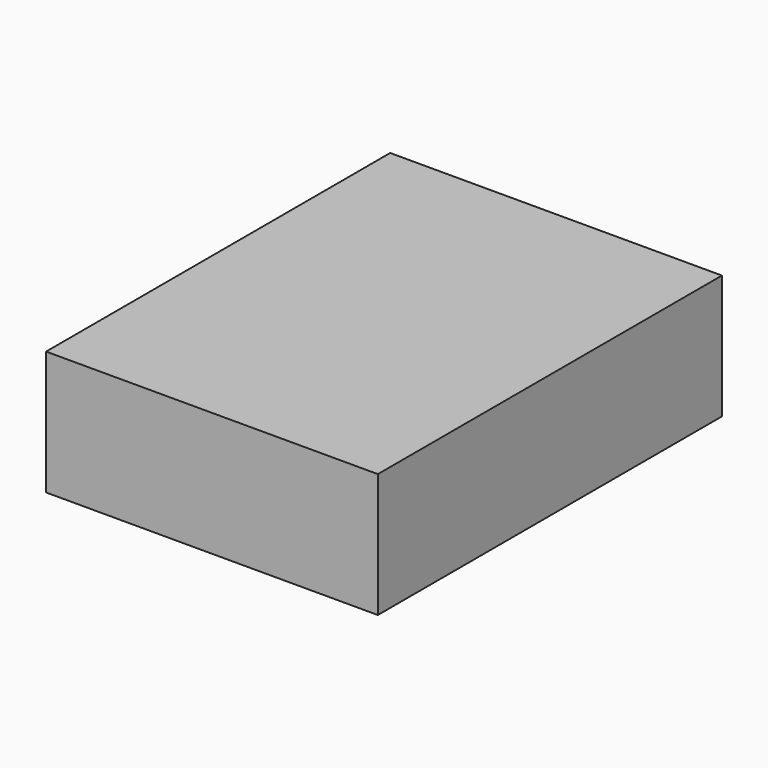
from build123d import *

# Parameters (mm, degrees)
F0_W     = 67.9279565811
F0_H     = 88.0647003651
F1_DEPTH = 25.4


# Not quite as in the source:
# - a feature of the source that left no trace in its solid (it failed there, or was rolled back) is left out


with BuildPart() as f1:
    # F0 (on Top) → F1 (new body)
    with BuildSketch(Plane.XY):
        Rectangle(F0_W, F0_H)
    extrude(amount=-F1_DEPTH)


solid = f1.part
